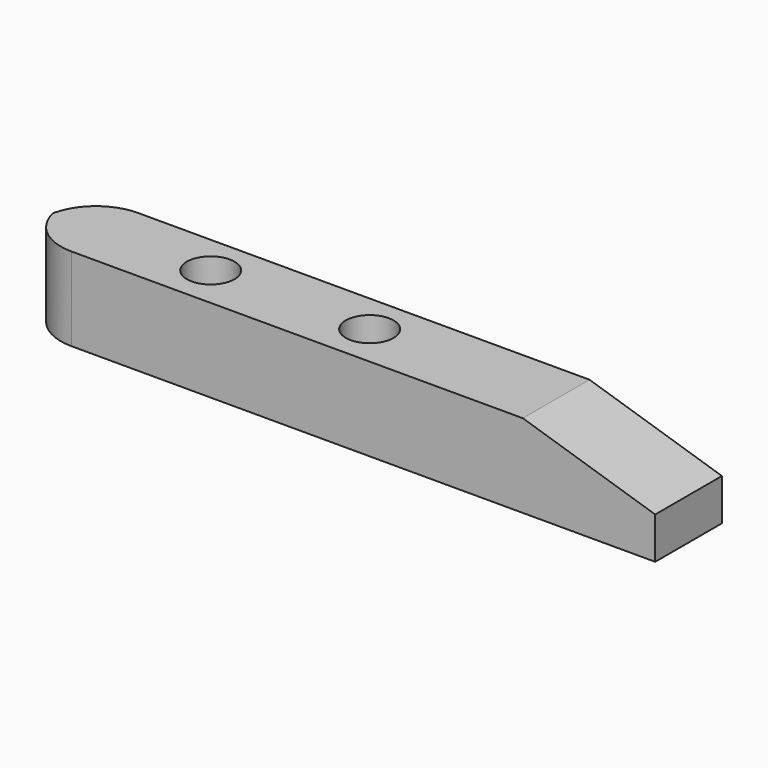
from build123d import *

# Parameters (mm, degrees)
F1_DEPTH    = 16.002
F3_D        = 9.144
F4_T1_DEPTH = 66.802


# Not quite as in the source:
# - a fillet or chamfer that OpenCascade refuses, or shapes differently, is made with other operations: its cross-section is extruded or revolved along the edge and cut away or added


with BuildPart() as f1:
    # F0 (on Front) → F1 (new body)
    with BuildSketch(Plane.XZ):
        Polygon((58.8562823832, 9.8717374111), (-37.9177176168, 9.8717374111), (-37.9177176168, -6.1302625889), (84.2562823832, -6.1302625889), (84.2562823832, 1.8707374111), align=None)
    extrude(amount=F1_DEPTH)

    # F3 (through all)
    with Locations(Plane.XY.offset(9.8717374111)):
        with Locations((-7.6279942878, -7.7707557939), (22.8794198483, -7.7707557939)):
            Hole(F3_D / 2)

    # F4: fillet of radius 10.16 on 2 edges, made by hand

    # F4_s2 → F4_t1 (cut)
    with BuildSketch(Plane.XY.offset(-31.5302625889)):
        with BuildLine():
            ThreePointArc((-27.7577176168, -16.002), (-34.9419225137, -13.0262048969), (-37.9177176168, -5.842))
            Line((-37.9177176168, -5.842), (-37.9177176168, -16.002))
            Line((-37.9177176168, -16.002), (-27.7577176168, -16.002))
        make_face()
        with BuildLine():
            ThreePointArc((-27.7577176168, 0), (-34.9419225137, -2.9757951031), (-37.9177176168, -10.16))
            Line((-37.9177176168, -10.16), (-37.9177176168, 0))
            Line((-37.9177176168, 0), (-27.7577176168, 0))
        make_face()
    extrude(amount=F4_T1_DEPTH, mode=Mode.SUBTRACT)


solid = f1.part
